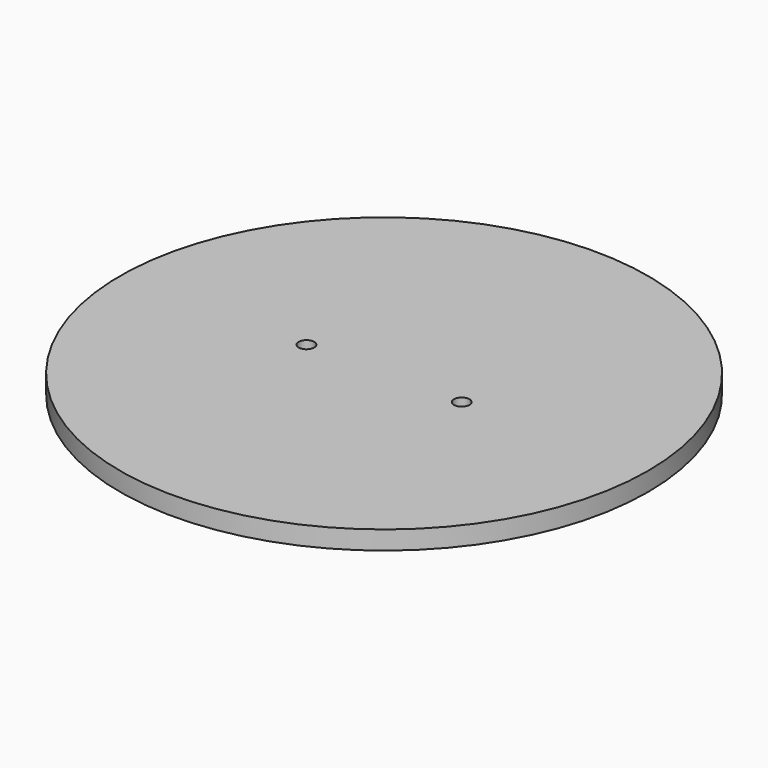
from build123d import *

# Parameters (mm, degrees)
F0_R     = 85
F1_DEPTH = 6
F3_D     = 5


# Not quite as in the source:
# - a feature of the source that left no trace in its solid (it failed there, or was rolled back) is left out


with BuildPart() as f1:
    # F0 (on Top) → F1 (new body)
    with BuildSketch(Plane.XY):
        Circle(F0_R)
    extrude(amount=F1_DEPTH)

    # F3 (through all)
    with Locations(Plane.XY.offset(6)):
        with Locations((-25, 0), (25, 0)):
            Hole(F3_D / 2)


solid = f1.part
